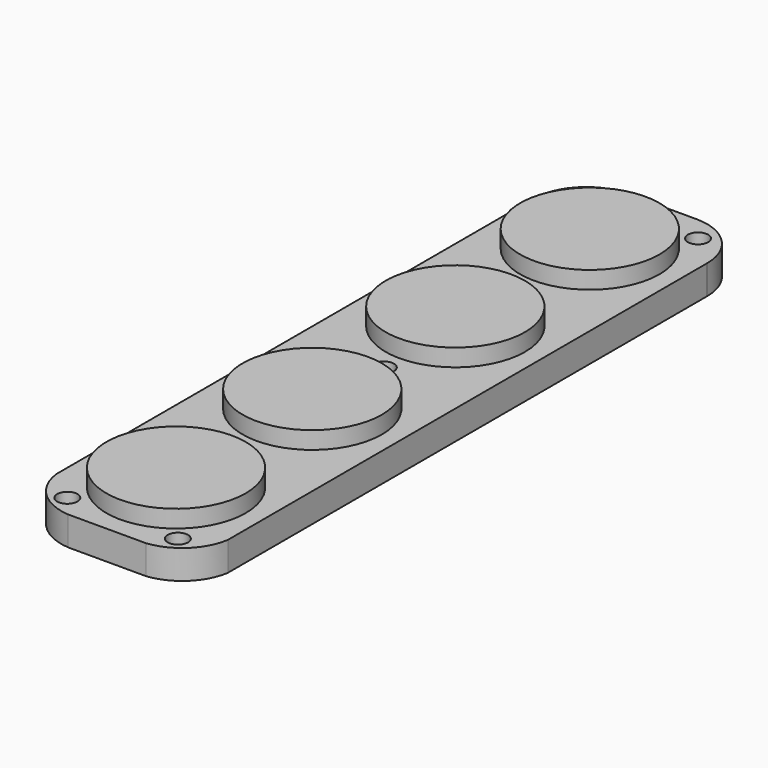
from build123d import *

# Parameters (mm, degrees)
F0_R          = 1.75
F0_R_2        = 1.25
F0_R_3        = 12
F1_DEPTH      = 5
F0_R_4        = 1
F2_START      = 3
F0_R_5        = 2
F2_DEPTH      = 2
F4_START      = 1.6
F4_DEPTH      = 3.4
F5_DEPTH      = 1.3
F5_DEPTH_BACK = 0.1
F6_START      = 5
F6_DEPTH      = 3


# Not quite as in the source:
# - a feature of the source that left no trace in its solid (it failed there, or was rolled back) is left out


with BuildPart() as f1:
    # F0 (on Top) → F1 (new body)
    with BuildSketch(Plane.XY):
        with BuildLine():
            Line((6.0037070689, 60.0215111673), (-5, 60.0215111673))
            Line((-5, 60.0215111673), (-6.7870675903, 60.0215111673))
            ThreePointArc((-6.7870675903, 60.0215111673), (-12.5859769766, 57.1353808627), (-15, 51.1245913098))
            Line((-15, 51.1245913098), (-15, 50.7903024554))
            Line((-15, 50.7903024554), (-15, -49.5038591325))
            Line((-15, -49.5038591325), (-15, -51.7690908138))
            ThreePointArc((-15, -51.7690908138), (-12.1695256151, -57.4125609321), (-6.4009595691, -59.9784888327))
            Line((-6.4009595691, -59.9784888327), (-5, -59.9784888327))
            Line((-5, -59.9784888327), (5, -59.9784888327))
            Line((5, -59.9784888327), (7.0074141379, -59.9784888327))
            ThreePointArc((7.0074141379, -59.9784888327), (12.2930504345, -57.5138166091), (15, -52.3480655233))
            Line((15, -52.3480655233), (15, -49.5038591325))
            Line((15, -49.5038591325), (15, 50.7903024554))
            Line((15, 50.7903024554), (15, 50.95497525))
            ThreePointArc((15, 50.95497525), (12.3454627339, 57.317569046), (6.0037070689, 60.0215111673))
        make_face()
        with Locations((-9.525, -56.2587864697)):
            Circle(F0_R, mode=Mode.SUBTRACT)
        with Locations((-9.525, -30.4671674967)):
            Circle(F0_R_2, mode=Mode.SUBTRACT)
        with Locations((0, -44.7514858243)):
            Circle(F0_R_3, mode=Mode.SUBTRACT)
        with Locations((-9.525, 0)):
            Circle(F0_R_2, mode=Mode.SUBTRACT)
        with Locations((0, -15.4157546586)):
            Circle(F0_R_3, mode=Mode.SUBTRACT)
        Circle(F0_R, mode=Mode.SUBTRACT)
        with Locations((9.525, -56.2587864697)):
            Circle(F0_R, mode=Mode.SUBTRACT)
        with Locations((9.525, -30.4671674967)):
            Circle(F0_R_2, mode=Mode.SUBTRACT)
        with Locations((9.525, 0)):
            Circle(F0_R_2, mode=Mode.SUBTRACT)
        with Locations((-9.525, 29.1974432766)):
            Circle(F0_R_2, mode=Mode.SUBTRACT)
        with Locations((0, 15.3948861798)):
            Circle(F0_R_3, mode=Mode.SUBTRACT)
        with Locations((-9.525, 55.7628124952)):
            Circle(F0_R, mode=Mode.SUBTRACT)
        with Locations((0, 44.3624239764)):
            Circle(F0_R_3, mode=Mode.SUBTRACT)
        with Locations((9.525, 29.1974432766)):
            Circle(F0_R_2, mode=Mode.SUBTRACT)
        with Locations((9.525, 55.7628124952)):
            Circle(F0_R, mode=Mode.SUBTRACT)
        with BuildLine():
            ThreePointArc((15, 50.7903024554), (15.0003704536, 50.8726388527), (15, 50.95497525))
            Line((15, 50.95497525), (15, 50.7903024554))
        make_face()
    extrude(amount=F1_DEPTH)



with BuildPart() as f1b:
    # F0 (on Top) → F1, piece 2 (new body)
    with BuildSketch(Plane.XY):
        with Locations((-9.525, 44.3624239764)):
            Circle(F0_R_4)
    extrude(amount=F1_DEPTH)


with BuildPart() as f1c:
    # F0 (on Top) → F1, piece 3 (new body)
    with BuildSketch(Plane.XY):
        with Locations((9.525, 44.3624239764)):
            Circle(F0_R_4)
    extrude(amount=F1_DEPTH)


with BuildPart() as f1d:
    # F0 (on Top) → F1, piece 4 (new body)
    with BuildSketch(Plane.XY):
        with Locations((9.525, 15.3948861798)):
            Circle(F0_R_4)
    extrude(amount=F1_DEPTH)


with BuildPart() as f1e:
    # F0 (on Top) → F1, piece 5 (new body)
    with BuildSketch(Plane.XY):
        with Locations((-9.525, 15.3948861798)):
            Circle(F0_R_4)
    extrude(amount=F1_DEPTH)


with BuildPart() as f1f:
    # F0 (on Top) → F1, piece 6 (new body)
    with BuildSketch(Plane.XY):
        with Locations((9.525, -15.4157546586)):
            Circle(F0_R_4)
    extrude(amount=F1_DEPTH)


with BuildPart() as f1g:
    # F0 (on Top) → F1, piece 7 (new body)
    with BuildSketch(Plane.XY):
        with Locations((-9.525, -15.4157546586)):
            Circle(F0_R_4)
    extrude(amount=F1_DEPTH)


with BuildPart() as f1h:
    # F0 (on Top) → F1, piece 8 (new body)
    with BuildSketch(Plane.XY):
        with Locations((9.525, -44.7514858243)):
            Circle(F0_R_4)
    extrude(amount=F1_DEPTH)


with BuildPart() as f1i:
    # F0 (on Top) → F1, piece 9 (new body)
    with BuildSketch(Plane.XY):
        with Locations((-9.525, -44.7514858243)):
            Circle(F0_R_4)
    extrude(amount=F1_DEPTH)


with BuildPart() as f1_1:
    add(f1.part)

    add(f1b.part)  # F2 merges F1b

    add(f1c.part)  # F2 merges F1c

    add(f1d.part)  # F2 merges F1d

    add(f1e.part)  # F2 merges F1e

    add(f1f.part)  # F2 merges F1f

    add(f1g.part)  # F2 merges F1g

    add(f1h.part)  # F2 merges F1h

    add(f1i.part)  # F2 merges F1i
    # F0 (on Top) → F2 (join)
    with BuildSketch(Plane.XY.offset(F2_START)):
        with Locations((0, 44.3624239764)):
            Circle(F0_R_3)
        with Locations((-9.525, 44.3624239764)):
            Circle(F0_R_5, mode=Mode.SUBTRACT)
        with Locations((9.525, 44.3624239764)):
            Circle(F0_R_5, mode=Mode.SUBTRACT)
        with Locations((0, 15.3948861798)):
            Circle(F0_R_3)
        with Locations((-9.525, 15.3948861798)):
            Circle(F0_R_5, mode=Mode.SUBTRACT)
        with Locations((9.525, 15.3948861798)):
            Circle(F0_R_5, mode=Mode.SUBTRACT)
        with Locations((0, -15.4157546586)):
            Circle(F0_R_3)
        with Locations((-9.525, -15.4157546586)):
            Circle(F0_R_5, mode=Mode.SUBTRACT)
        with Locations((9.525, -15.4157546586)):
            Circle(F0_R_5, mode=Mode.SUBTRACT)
        with Locations((0, -44.7514858243)):
            Circle(F0_R_3)
        with Locations((-9.525, -44.7514858243)):
            Circle(F0_R_5, mode=Mode.SUBTRACT)
        with Locations((9.525, -44.7514858243)):
            Circle(F0_R_5, mode=Mode.SUBTRACT)
        with Locations((9.525, 44.3624239764)):
            Circle(F0_R_5)
        with Locations((9.525, 44.3624239764)):
            Circle(F0_R_4, mode=Mode.SUBTRACT)
        with Locations((-9.525, 44.3624239764)):
            Circle(F0_R_5)
        with Locations((-9.525, 44.3624239764)):
            Circle(F0_R_4, mode=Mode.SUBTRACT)
        with Locations((9.525, 15.3948861798)):
            Circle(F0_R_5)
        with Locations((9.525, 15.3948861798)):
            Circle(F0_R_4, mode=Mode.SUBTRACT)
        with Locations((-9.525, 15.3948861798)):
            Circle(F0_R_5)
        with Locations((-9.525, 15.3948861798)):
            Circle(F0_R_4, mode=Mode.SUBTRACT)
        with Locations((9.525, -15.4157546586)):
            Circle(F0_R_5)
        with Locations((9.525, -15.4157546586)):
            Circle(F0_R_4, mode=Mode.SUBTRACT)
        with Locations((-9.525, -15.4157546586)):
            Circle(F0_R_5)
        with Locations((-9.525, -15.4157546586)):
            Circle(F0_R_4, mode=Mode.SUBTRACT)
        with Locations((9.525, -44.7514858243)):
            Circle(F0_R_5)
        with Locations((9.525, -44.7514858243)):
            Circle(F0_R_4, mode=Mode.SUBTRACT)
        with Locations((-9.525, -44.7514858243)):
            Circle(F0_R_5)
        with Locations((-9.525, -44.7514858243)):
            Circle(F0_R_4, mode=Mode.SUBTRACT)
        with Locations((-9.525, -30.4671674967)):
            Circle(F0_R_2)
        with Locations((9.525, -30.4671674967)):
            Circle(F0_R_2)
        with Locations((9.525, 0)):
            Circle(F0_R_2)
        with Locations((-9.525, 0)):
            Circle(F0_R_2)
        with Locations((-9.525, 29.1974432766)):
            Circle(F0_R_2)
        with Locations((9.525, 29.1974432766)):
            Circle(F0_R_2)
        with Locations((9.525, 44.3624239764)):
            Circle(F0_R_4)
        with Locations((-9.525, 44.3624239764)):
            Circle(F0_R_4)
        with Locations((9.525, 15.3948861798)):
            Circle(F0_R_4)
        with Locations((-9.525, 15.3948861798)):
            Circle(F0_R_4)
        with Locations((9.525, -15.4157546586)):
            Circle(F0_R_4)
        with Locations((-9.525, -15.4157546586)):
            Circle(F0_R_4)
        with Locations((9.525, -44.7514858243)):
            Circle(F0_R_4)
        with Locations((-9.525, -44.7514858243)):
            Circle(F0_R_4)
    extrude(amount=F2_DEPTH)

    # F0 (on Top) → F4 (join)
    with BuildSketch(Plane.XY.offset(F4_START)):
        with Locations((9.525, 44.3624239764)):
            Circle(F0_R_5)
        with Locations((9.525, 44.3624239764)):
            Circle(F0_R_4, mode=Mode.SUBTRACT)
        with Locations((-9.525, 44.3624239764)):
            Circle(F0_R_5)
        with Locations((-9.525, 44.3624239764)):
            Circle(F0_R_4, mode=Mode.SUBTRACT)
        with Locations((9.525, 15.3948861798)):
            Circle(F0_R_5)
        with Locations((9.525, 15.3948861798)):
            Circle(F0_R_4, mode=Mode.SUBTRACT)
        with Locations((-9.525, 15.3948861798)):
            Circle(F0_R_5)
        with Locations((-9.525, 15.3948861798)):
            Circle(F0_R_4, mode=Mode.SUBTRACT)
        with Locations((9.525, -15.4157546586)):
            Circle(F0_R_5)
        with Locations((9.525, -15.4157546586)):
            Circle(F0_R_4, mode=Mode.SUBTRACT)
        with Locations((-9.525, -15.4157546586)):
            Circle(F0_R_5)
        with Locations((-9.525, -15.4157546586)):
            Circle(F0_R_4, mode=Mode.SUBTRACT)
        with Locations((9.525, -44.7514858243)):
            Circle(F0_R_5)
        with Locations((9.525, -44.7514858243)):
            Circle(F0_R_4, mode=Mode.SUBTRACT)
        with Locations((-9.525, -44.7514858243)):
            Circle(F0_R_5)
        with Locations((-9.525, -44.7514858243)):
            Circle(F0_R_4, mode=Mode.SUBTRACT)
    extrude(amount=F4_DEPTH)

    # F0 (on Top) → F5 (cut, two sides)
    with BuildSketch(Plane.XY) as f5_sk:
        with Locations((9.525, -56.2587864697)):
            Circle(F0_R)
        with Locations((-9.525, -56.2587864697)):
            Circle(F0_R)
        with Locations((-9.525, -30.4671674967)):
            Circle(F0_R_2)
        with Locations((9.525, -30.4671674967)):
            Circle(F0_R_2)
        with Locations((9.525, 0)):
            Circle(F0_R_2)
        with Locations((-9.525, 0)):
            Circle(F0_R_2)
        with Locations((9.525, 29.1974432766)):
            Circle(F0_R_2)
        with Locations((-9.525, 29.1974432766)):
            Circle(F0_R_2)
        with Locations((9.525, 55.7628124952)):
            Circle(F0_R)
        with Locations((-9.525, 55.7628124952)):
            Circle(F0_R)
    extrude(amount=F5_DEPTH, mode=Mode.SUBTRACT)
    extrude(f5_sk.sketch, amount=-F5_DEPTH_BACK, mode=Mode.SUBTRACT)

    # F0 (on Top) → F6 (join)
    with BuildSketch(Plane.XY.offset(F6_START)):
        with Locations((0, 44.3624239764)):
            Circle(F0_R_3)
        with Locations((-9.525, 44.3624239764)):
            Circle(F0_R_5, mode=Mode.SUBTRACT)
        with Locations((9.525, 44.3624239764)):
            Circle(F0_R_5, mode=Mode.SUBTRACT)
        with Locations((0, 15.3948861798)):
            Circle(F0_R_3)
        with Locations((-9.525, 15.3948861798)):
            Circle(F0_R_5, mode=Mode.SUBTRACT)
        with Locations((9.525, 15.3948861798)):
            Circle(F0_R_5, mode=Mode.SUBTRACT)
        with Locations((0, -15.4157546586)):
            Circle(F0_R_3)
        with Locations((-9.525, -15.4157546586)):
            Circle(F0_R_5, mode=Mode.SUBTRACT)
        with Locations((9.525, -15.4157546586)):
            Circle(F0_R_5, mode=Mode.SUBTRACT)
        with Locations((0, -44.7514858243)):
            Circle(F0_R_3)
        with Locations((-9.525, -44.7514858243)):
            Circle(F0_R_5, mode=Mode.SUBTRACT)
        with Locations((9.525, -44.7514858243)):
            Circle(F0_R_5, mode=Mode.SUBTRACT)
        with Locations((-9.525, -44.7514858243)):
            Circle(F0_R_5)
        with Locations((-9.525, -44.7514858243)):
            Circle(F0_R_4, mode=Mode.SUBTRACT)
        with Locations((9.525, -44.7514858243)):
            Circle(F0_R_5)
        with Locations((9.525, -44.7514858243)):
            Circle(F0_R_4, mode=Mode.SUBTRACT)
        with Locations((-9.525, -15.4157546586)):
            Circle(F0_R_5)
        with Locations((-9.525, -15.4157546586)):
            Circle(F0_R_4, mode=Mode.SUBTRACT)
        with Locations((9.525, -15.4157546586)):
            Circle(F0_R_5)
        with Locations((9.525, -15.4157546586)):
            Circle(F0_R_4, mode=Mode.SUBTRACT)
        with Locations((-9.525, 15.3948861798)):
            Circle(F0_R_5)
        with Locations((-9.525, 15.3948861798)):
            Circle(F0_R_4, mode=Mode.SUBTRACT)
        with Locations((9.525, 15.3948861798)):
            Circle(F0_R_5)
        with Locations((9.525, 15.3948861798)):
            Circle(F0_R_4, mode=Mode.SUBTRACT)
        with Locations((-9.525, 44.3624239764)):
            Circle(F0_R_5)
        with Locations((-9.525, 44.3624239764)):
            Circle(F0_R_4, mode=Mode.SUBTRACT)
        with Locations((9.525, 44.3624239764)):
            Circle(F0_R_5)
        with Locations((9.525, 44.3624239764)):
            Circle(F0_R_4, mode=Mode.SUBTRACT)
        with Locations((-9.525, -44.7514858243)):
            Circle(F0_R_4)
        with Locations((9.525, -44.7514858243)):
            Circle(F0_R_4)
        with Locations((-9.525, -15.4157546586)):
            Circle(F0_R_4)
        with Locations((9.525, -15.4157546586)):
            Circle(F0_R_4)
        with Locations((-9.525, 15.3948861798)):
            Circle(F0_R_4)
        with Locations((9.525, 15.3948861798)):
            Circle(F0_R_4)
        with Locations((-9.525, 44.3624239764)):
            Circle(F0_R_4)
        with Locations((9.525, 44.3624239764)):
            Circle(F0_R_4)
    extrude(amount=F6_DEPTH)


solid = f1_1.part
